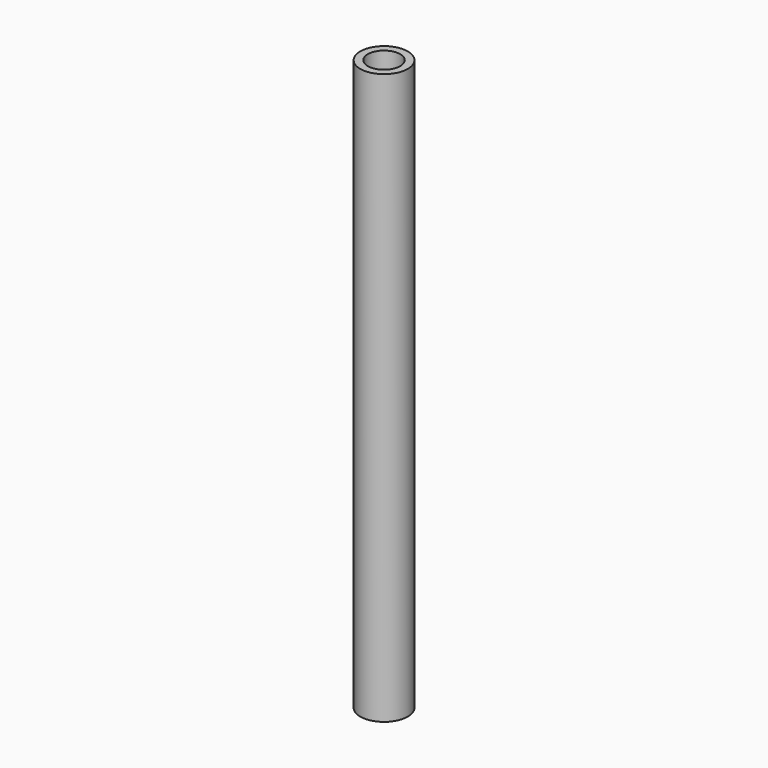
from build123d import *

# Parameters (mm, degrees)
F0_R     = 38.1
F0_R_2   = 22.225
F1_DEPTH = 914.4
F3_R     = 26
F3_R_2   = 22.225
F4_DEPTH = 152.4
F5_R     = 24.09825
F6_DEPTH = 6.35


# Not quite as in the source:
# - a feature names something its author has since deleted; it is built from what else it names


with BuildPart() as f1:
    # F0 (on Top) → F1 (new body)
    with BuildSketch(Plane.XY):
        Circle(F0_R)
        Circle(F0_R_2, mode=Mode.SUBTRACT)
    extrude(amount=F1_DEPTH)

    # F3 (on face) → F4 (cut)
    with BuildSketch(Plane.XY.offset(914.4)):
        Circle(F3_R)
        Circle(F3_R_2, mode=Mode.SUBTRACT)
    extrude(amount=-F4_DEPTH, mode=Mode.SUBTRACT)

    # F5 (on face) → F6 (cut)
    with BuildSketch(Plane.XY.offset(762)):
        Circle(F5_R)
    extrude(amount=-F6_DEPTH, mode=Mode.SUBTRACT)


solid = f1.part
